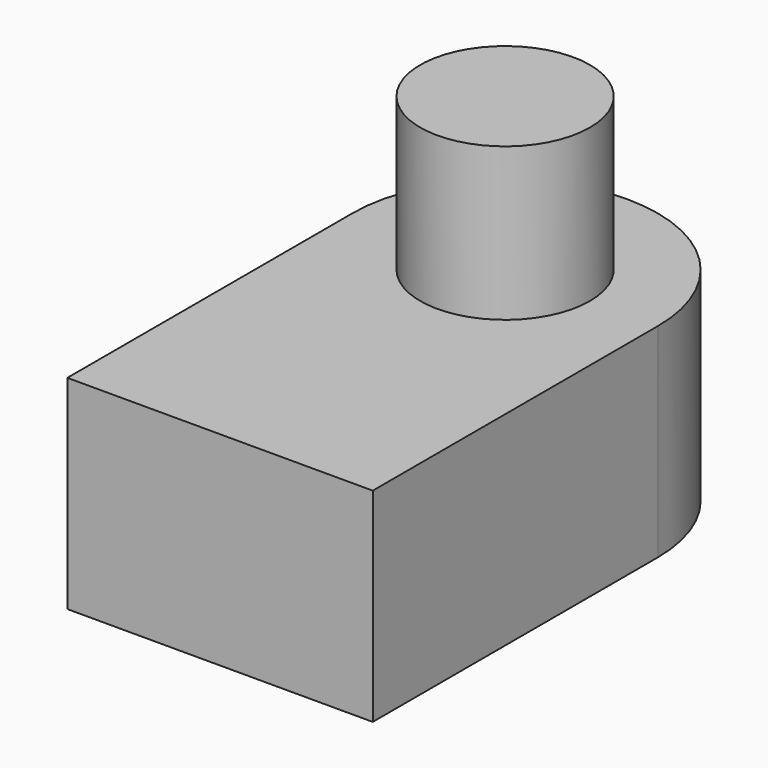
from build123d import *

# Parameters (mm, degrees)
F0_W     = 9
F0_H     = 15
F1_DEPTH = 6
F2_R     = 2.5
F3_DEPTH = 4.5
F4_R     = 4.49999


# Not quite as in the source:
# - a fillet or chamfer is up to 0.001 mm smaller than in the source, because OpenCascade refuses the exact size


with BuildPart() as f1:
    # F0 (on Top) → F1 (new body)
    with BuildSketch(Plane.XY):
        Rectangle(F0_W, F0_H)
    extrude(amount=F1_DEPTH)

    # F2 (on face) → F3 (join)
    with BuildSketch(Plane.XY.offset(6)):
        with Locations((0, 3)):
            Circle(F2_R)
    extrude(amount=F3_DEPTH)

    # F4 (radius 4.5 in the source; OpenCascade refuses exactly that, so slightly less here)
    f4_edges = [f1.edges().sort_by_distance(p)[0] for p in [
        (-4.5, 7.5, 3),
        (4.5, 7.5, 3),
    ]]
    fillet(f4_edges, radius=F4_R)


solid = f1.part
